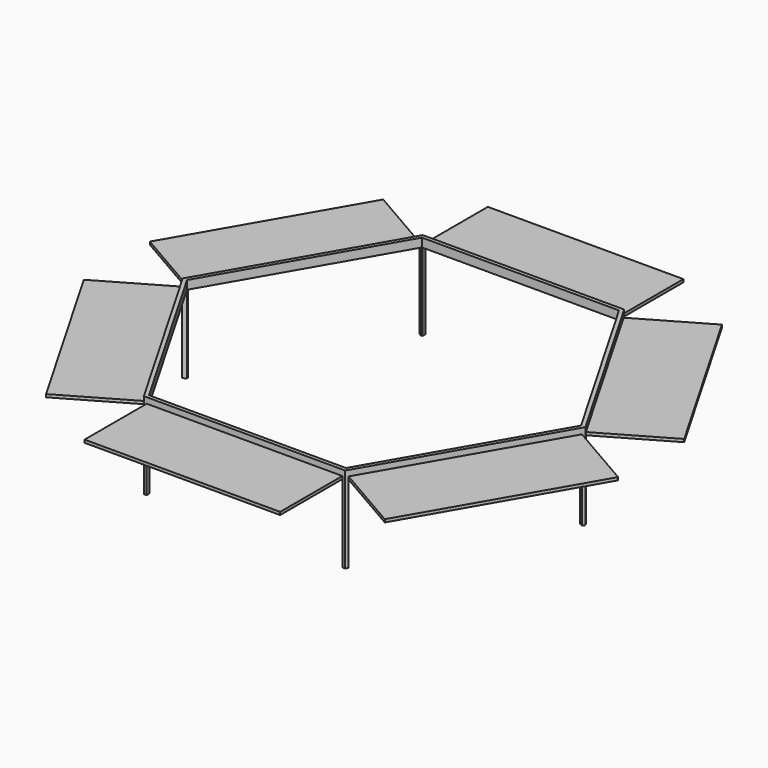
from build123d import *

# Parameters (mm, degrees)
F1_DEPTH  = 3000
F2_W      = 6800
F2_H      = 2700
F3_DEPTH  = 15155.4455662277
F4_W      = 6800
F4_H      = 2700
F5_DEPTH  = 15155.4455662277
F6_W      = 6800
F6_H      = 2700
F7_DEPTH  = 12124.3566529821
F8_W      = 6800
F8_H      = 100
F9_DEPTH  = 2700
F10_W     = 6800
F10_H     = 100
F11_DEPTH = 2700
F12_W     = 6800
F12_H     = 100
F13_DEPTH = 2700
F14_W     = 6800
F14_H     = 100
F15_DEPTH = 2700
F16_W     = 6800
F16_H     = 100
F17_DEPTH = 2700
F18_W     = 6800
F18_H     = 100
F19_DEPTH = 2700


with BuildPart() as f1:
    # F0 (on Top) → F1 (new body)
    with BuildSketch(Plane.XY):
        Polygon((3500, -6062.1778264911), (7000, 0), (3500, 6062.1778264911), (-3500, 6062.1778264911), (-7000, 0), (-3500, -6062.1778264911), align=None)
        Polygon((3425, 5932.2740159234), (6850, 0), (3425, -5932.2740159234), (-3425, -5932.2740159234), (-6850, 0), (-3425, 5932.2740159234), align=None, mode=Mode.SUBTRACT)
    extrude(amount=F1_DEPTH)

    # F2 (on face) → F3 (cut, through all)
    with BuildSketch(Plane(origin=(-5250, -3031.0889132455, 0), x_dir=(0.5, -0.8660254038, 0), z_dir=(-0.8660254038, -0.5, 0))):
        with Locations((0, 1350)):
            Rectangle(F2_W, F2_H)
    extrude(amount=-F3_DEPTH, mode=Mode.SUBTRACT)

    # F4 (on face) → F5 (cut, through all)
    with BuildSketch(Plane(origin=(-5250, 3031.0889132455, 0), x_dir=(-0.5, -0.8660254038, 0), z_dir=(-0.8660254038, 0.5, 0))):
        with Locations((0, 1350)):
            Rectangle(F4_W, F4_H)
    extrude(amount=-F5_DEPTH, mode=Mode.SUBTRACT)

    # F6 (on face) → F7 (cut, through all)
    with BuildSketch(Plane(origin=(0, 6062.1778264911, 0), x_dir=(-1, 0, 0), z_dir=(0, 1, 0))):
        with Locations((0, 1350)):
            Rectangle(F6_W, F6_H)
    extrude(amount=-F7_DEPTH, mode=Mode.SUBTRACT)

    # F8 (on face) → F9 (join)
    with BuildSketch(Plane(origin=(0, 6062.1778264911, 0), x_dir=(-1, 0, 0), z_dir=(0, 1, 0))):
        with Locations((0, 2750)):
            Rectangle(F8_W, F8_H)
    extrude(amount=F9_DEPTH)

    # F10 (on face) → F11 (join)
    with BuildSketch(Plane(origin=(5250, 3031.0889132455, 0), x_dir=(-0.5, 0.8660254038, 0), z_dir=(0.8660254038, 0.5, 0))):
        with Locations((0, 2750)):
            Rectangle(F10_W, F10_H)
    extrude(amount=F11_DEPTH)

    # F12 (on face) → F13 (join)
    with BuildSketch(Plane(origin=(5250, -3031.0889132455, 0), x_dir=(0.5, 0.8660254038, 0), z_dir=(0.8660254038, -0.5, 0))):
        with Locations((0, 2750)):
            Rectangle(F12_W, F12_H)
    extrude(amount=F13_DEPTH)

    # F14 (on face) → F15 (join)
    with BuildSketch(Plane.XZ.offset(6062.1778264911)):
        with Locations((0, 2750)):
            Rectangle(F14_W, F14_H)
    extrude(amount=F15_DEPTH)

    # F16 (on face) → F17 (join)
    with BuildSketch(Plane(origin=(-5250, -3031.0889132455, 0), x_dir=(0.5, -0.8660254038, 0), z_dir=(-0.8660254038, -0.5, 0))):
        with Locations((0, 2750)):
            Rectangle(F16_W, F16_H)
    extrude(amount=F17_DEPTH)

    # F18 (on face) → F19 (join)
    with BuildSketch(Plane(origin=(-5250, 3031.0889132455, 0), x_dir=(-0.5, -0.8660254038, 0), z_dir=(-0.8660254038, 0.5, 0))):
        with Locations((0, 2750)):
            Rectangle(F18_W, F18_H)
    extrude(amount=F19_DEPTH)


solid = f1.part
